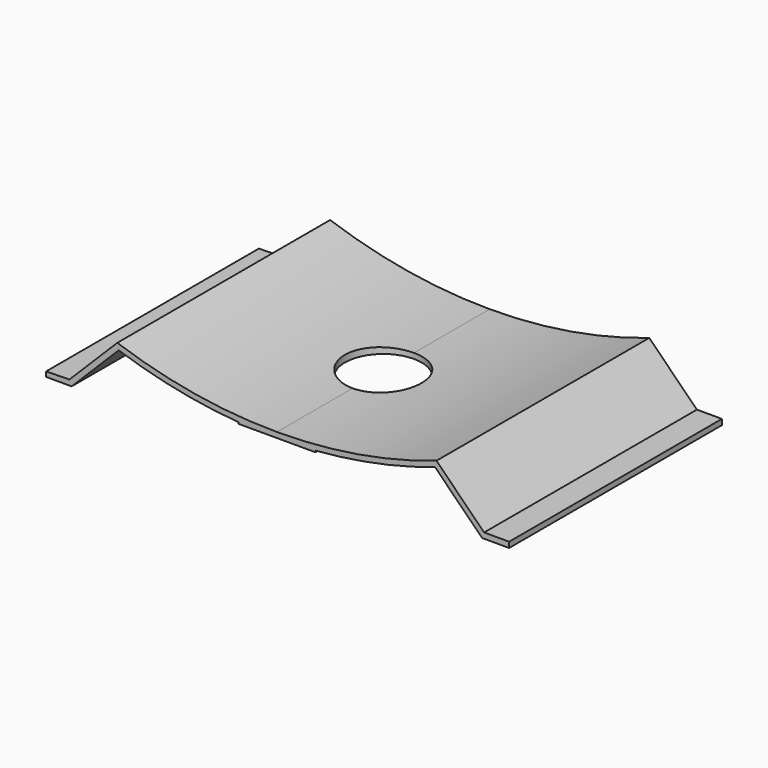
from build123d import *

# Parameters (mm, degrees)
F0_W        = 10
F0_H        = 5
F1_DEPTH    = 1
F2_T1_DEPTH = 15.2867319519
F4_DEPTH    = 25
F6_DEPTH    = 5
F8_DEPTH    = 5
F9_R        = 0.72
F10_DEPTH   = 1


# Not quite as in the source:
# - a fillet or chamfer that OpenCascade refuses, or shapes differently, is made with other operations: its cross-section is extruded or revolved along the edge and cut away or added


with BuildPart() as f1:
    # F0 (on Top) → F1 (new body)
    with BuildSketch(Plane.XY):
        with Locations((5, 2.5)):
            Rectangle(F0_W, F0_H)
    extrude(amount=F1_DEPTH)

    # F2: chamfer of 2 on 2 edges, made by hand

    # F2_s2 → F2_t1 (cut)
    with BuildSketch(Plane.XZ.offset(-10.1433659759)):
        Polygon((0, -1), (2, 1), (0, 1), align=None)
        Polygon((10, -1), (8, 1), (10, 1), align=None)
    extrude(amount=F2_T1_DEPTH, mode=Mode.SUBTRACT)

    # F3 (on face) → F4 (cut)
    with BuildSketch(Plane.XZ):
        with BuildLine():
            Line((5, 0.5), (5, 1))
            Line((5, 1), (2, 1))
            ThreePointArc((2, 1), (3.4793093674, 0.6258562046), (5, 0.5))
        make_face()
        with BuildLine():
            Line((8, 1), (5, 1))
            Line((5, 1), (5, 0.5))
            ThreePointArc((5, 0.5), (6.5206906326, 0.6258562046), (8, 1))
        make_face()
        with BuildLine():
            Line((1.1414213562, 0), (8.8585786438, 0))
            Line((8.8585786438, 0), (7.9732451927, 0.8853334511))
            ThreePointArc((7.9732451927, 0.8853334511), (5, 0.4), (2.0267548073, 0.8853334511))
            Line((2.0267548073, 0.8853334511), (1.1414213562, 0))
        make_face()
    extrude(amount=-F4_DEPTH, mode=Mode.SUBTRACT)

    # F5 (on face) → F6 (join)
    with BuildSketch(Plane.XZ):
        Polygon((8.8956828495, 0.1043171505), (9, 0), (9.3658352271, 0), (9.3658352271, 0.1043171505), align=None)
        Polygon((0.6632895378, 0), (1, 0), (1.1006881325, 0.1006881325), (0.6614453159, 0.0918707301), align=None)
    extrude(amount=-F6_DEPTH)

    # F7 (on face) → F8 (join)
    with BuildSketch(Plane.XZ):
        with BuildLine():
            Line((4.275, 0.4), (5, 0.4))
            ThreePointArc((5, 0.4), (4.6372268408, 0.4070403172), (4.275, 0.4281506663))
            Line((4.275, 0.4281506663), (4.275, 0.4))
        make_face()
        with BuildLine():
            ThreePointArc((5.725, 0.4281506663), (5.3627731592, 0.4070403172), (5, 0.4))
            Line((5, 0.4), (5.725, 0.4))
            Line((5.725, 0.4), (5.725, 0.4281506663))
        make_face()
    extrude(amount=-F8_DEPTH)

    # F9 (on face) → F10 (cut)
    with BuildSketch(Plane(origin=(0, 0, 0.4), x_dir=(1, 0, 0), z_dir=(0, 0, -1))):
        with Locations((5, -2.5)):
            Circle(F9_R)
    extrude(amount=-F10_DEPTH, mode=Mode.SUBTRACT)


solid = f1.part
